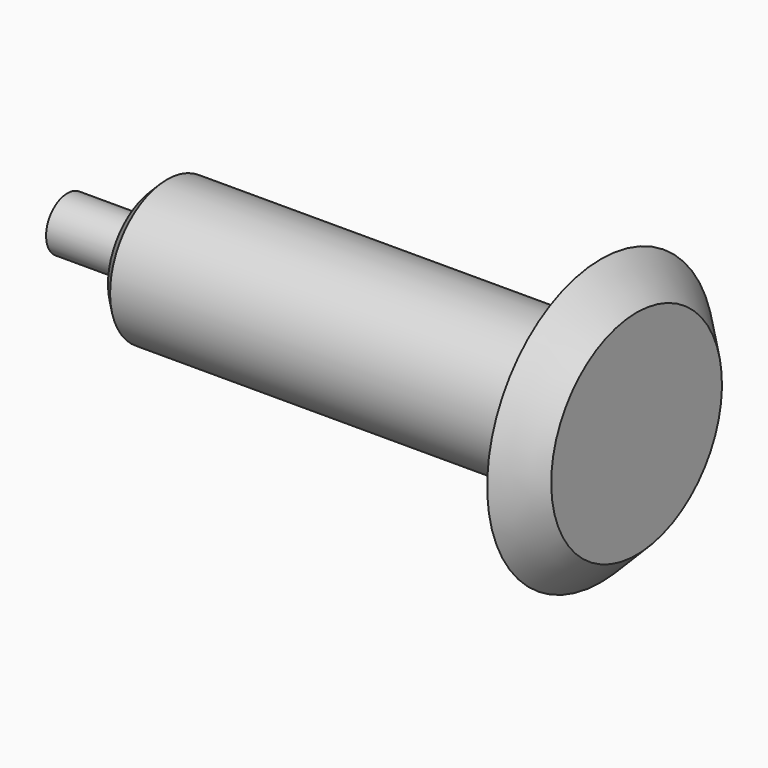
from build123d import *

# Parameters (mm, degrees)
F0_W     = 25
F0_H     = 7.5
F2_SIZE2 = 3
F2_SIZE  = 3
F3_SIZE2 = 9.99999
F3_SIZE  = 9.99999


# Not quite as in the source:
# - a fillet or chamfer is up to 0.001 mm smaller than in the source, because OpenCascade refuses the exact size


with BuildPart() as f1:
    # F0 (on Front) → F1 (revolve)
    with BuildSketch(Plane.XZ):
        with Locations((12.5, 11.25)):
            Rectangle(F0_W, F0_H)
        Polygon((25, 15), (25, 7.5), (140, 7.5), (140, 27.5), (25, 27.5), align=None)
        Polygon((140, 27.5), (140, 7.5), (150, 7.5), (150, 37.5), align=None)
        Polygon((150, 37.5), (150, 7.5), (160, 7.5), (160, 47.5), (150, 47.5), align=None)
    revolve(axis=Axis((80, 0, 7.5), (1, 0, 0)))

    # F2
    f2_edges = [f1.edges().sort_by_distance(p)[0] for p in [
        (25, 0, -12.5),
    ]]
    chamfer(f2_edges, length=F2_SIZE, length2=F2_SIZE2)

    # F3 (size 10 and 10 in the source; OpenCascade refuses exactly that, so slightly less here)
    f3_edges = [f1.edges().sort_by_distance(p)[0] for p in [
        (160, 0, -32.5),
    ]]
    chamfer(f3_edges, length=F3_SIZE, length2=F3_SIZE2)


solid = f1.part
